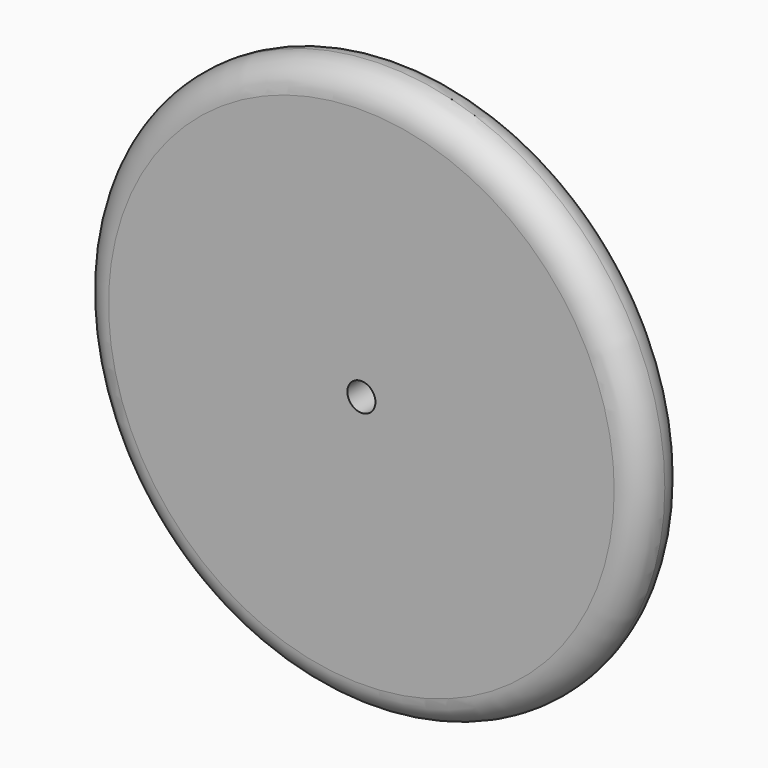
from build123d import *

# Parameters (mm, degrees)
F0_R     = 12.7
F1_DEPTH = 2.54
F2_R     = 0.635
F3_DEPTH = 25.4
F4_R     = 1.26999


# Not quite as in the source:
# - a fillet or chamfer is up to 0.001 mm smaller than in the source, because OpenCascade refuses the exact size


with BuildPart() as f1:
    # F0 (on Front) → F1 (new body)
    with BuildSketch(Plane.XZ):
        Circle(F0_R)
    extrude(amount=F1_DEPTH)

    # F2 (on face) → F3 (cut)
    with BuildSketch(Plane.XZ.offset(2.54)):
        Circle(F2_R)
    extrude(amount=-F3_DEPTH, mode=Mode.SUBTRACT)

    # F4 (radius 1.27 in the source; OpenCascade refuses exactly that, so slightly less here)
    f4_edges = [f1.edges().sort_by_distance(p)[0] for p in [
        (-12.7, -2.54, 0),
        (-12.7, 0, 0),
    ]]
    fillet(f4_edges, radius=F4_R)


solid = f1.part
